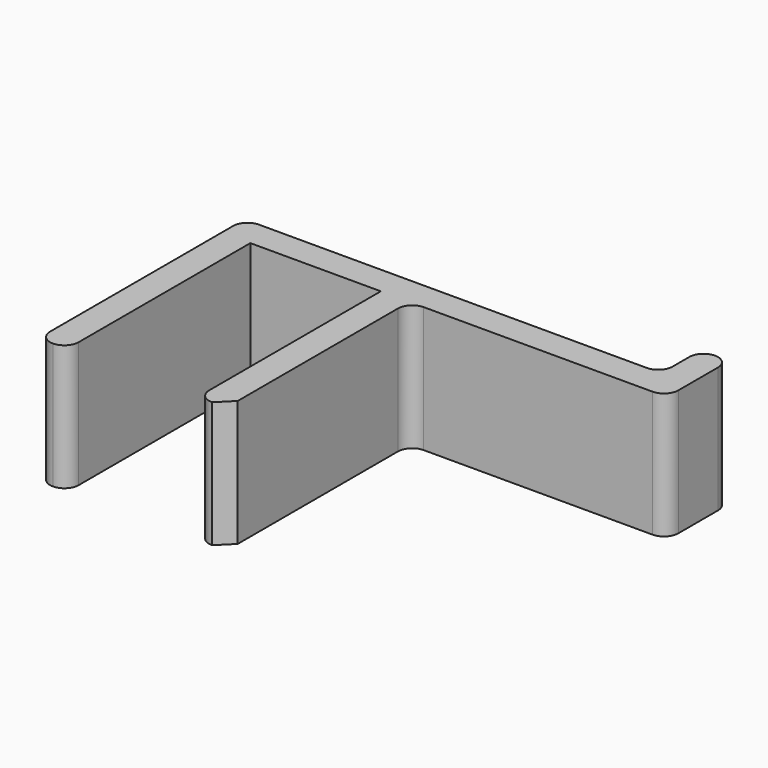
from build123d import *

# Parameters (mm, degrees)
F1_DEPTH = 22
F2_R     = 2.49999
F3_SIZE  = 2.5
F4_R     = 2.49999


# Not quite as in the source:
# - a fillet or chamfer is up to 0.001 mm smaller than in the source, because OpenCascade refuses the exact size


with BuildPart() as f1:
    # F0 (on Top) → F1 (new body)
    with BuildSketch(Plane.XY):
        Polygon((0, -40), (0, 0), (22.8, 0), (22.8, -40), (27.8, -40), (27.8, 0), (72.8, 0), (72.8, 13.6540349229), (67.8, 13.6540349229), (67.8, 5), (-5, 5), (-5, -40), align=None)
    extrude(amount=F1_DEPTH)

    # F2 (radius 2.5 in the source; OpenCascade refuses exactly that, so slightly less here)
    f2_edges = [f1.edges().sort_by_distance(p)[0] for p in [
        (72.8, 0, 11),
        (27.8, 0, 11),
        (67.8, 5, 11),
        (67.8, 13.654035, 11),
        (72.8, 13.654035, 11),
        (-5, 5, 11),
        (-5, -40, 11),
        (0, -40, 11),
    ]]
    fillet(f2_edges, radius=F2_R)

    # F3
    f3_edges = [f1.edges().sort_by_distance(p)[0] for p in [
        (27.8, -40, 11),
    ]]
    chamfer(f3_edges, length=F3_SIZE)

    # F4 (radius 2.5 in the source; OpenCascade refuses exactly that, so slightly less here)
    f4_edges = [f1.edges().sort_by_distance(p)[0] for p in [
        (22.8, -40, 11),
    ]]
    fillet(f4_edges, radius=F4_R)


solid = f1.part
